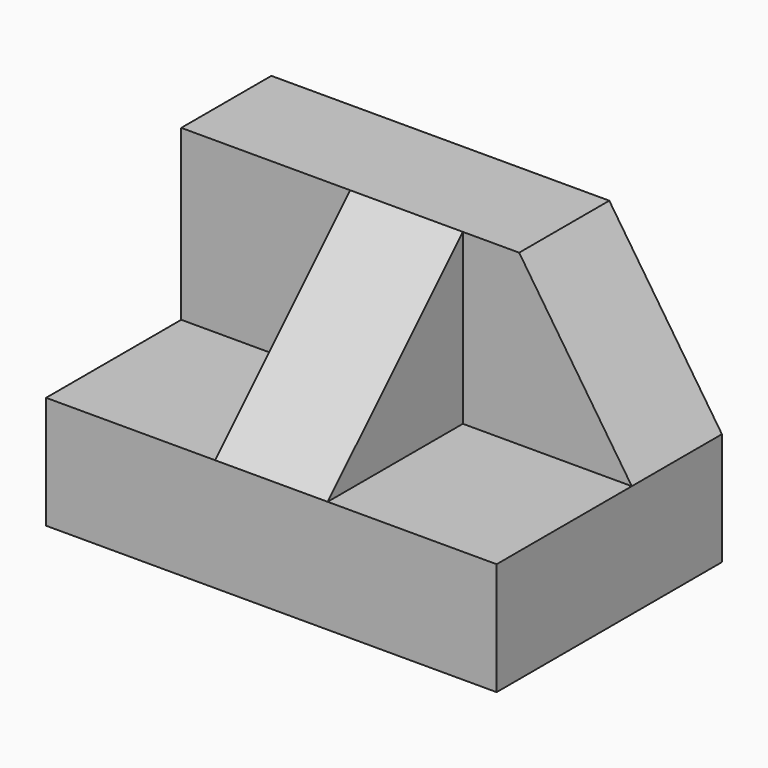
from build123d import *

# Parameters (mm, degrees)
F0_W     = 50.8
F0_H     = 31.75
F1_DEPTH = 31.75
F2_W     = 19.05
F2_H     = 19.05
F3_DEPTH = 19.05
F4_W     = 19.05
F4_H     = 19.05
F5_DEPTH = 19.05
F7_DEPTH = 25.4
F9_DEPTH = 25.4


# Not quite as in the source:
# - a feature names something its author has since deleted; it is built from what else it names


with BuildPart() as f1:
    # F0 (on Front) → F1 (new body)
    with BuildSketch(Plane.XZ):
        with Locations((25.4, 15.875)):
            Rectangle(F0_W, F0_H)
    extrude(amount=F1_DEPTH)

    # F2 (on face) → F3 (cut)
    with BuildSketch(Plane.XZ.offset(31.75)):
        with Locations((41.275, 22.225)):
            Rectangle(F2_W, F2_H)
    extrude(amount=-F3_DEPTH, mode=Mode.SUBTRACT)

    # F4 (on face) → F5 (cut)
    with BuildSketch(Plane.XZ.offset(31.75)):
        with Locations((9.525, 22.225)):
            Rectangle(F4_W, F4_H)
    extrude(amount=-F5_DEPTH, mode=Mode.SUBTRACT)

    # F6 (on face) → F7 (cut)
    with BuildSketch(Plane.YZ.offset(31.75)):
        Polygon((-31.75, 31.75), (-31.75, 12.7), (-12.7, 31.75), align=None)
    extrude(amount=-F7_DEPTH, mode=Mode.SUBTRACT)

    # F8 (on face) → F9 (cut)
    with BuildSketch(Plane.XZ.offset(12.7)):
        Polygon((50.8, 31.75), (38.1, 31.75), (50.8, 12.7), align=None)
    extrude(amount=-F9_DEPTH, mode=Mode.SUBTRACT)


solid = f1.part
